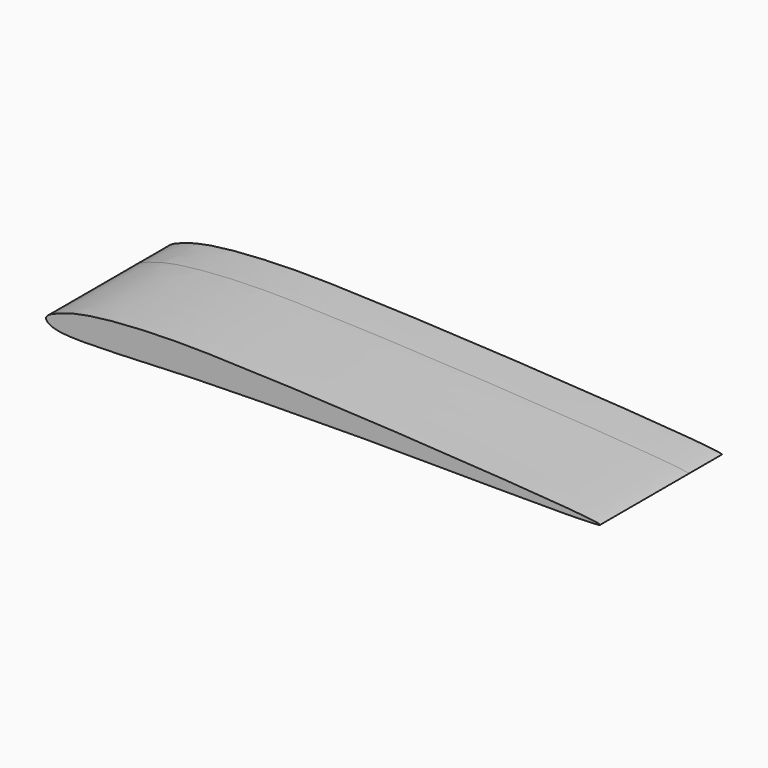
from build123d import *

# Parameters (mm, degrees)
F1_DEPTH = 20
F2_DEPTH = 7.5


with BuildPart() as f1:
    # F0 (on Front) → F1 (new body)
    with BuildSketch(Plane.XZ):
        with BuildLine():
            add(Edge.make_bspline(
                [(50.3091172778, -1.1656129636), (50.1718635236, -0.614292774), (8.6569150114, 1.9894121194), (-12.2185501878, 2.7626849393), (-26.6473375965, 3.249698923), (-38.2423795462, 2.6501887814), (-44.081300152, 1.7253239287), (-46.8139447574, 0.9123113702), (-50.2879633949, -0.4217517299), (-48.9166705509, -2.2301634685), (-42.4139489162, -2.6824339621), (-26.2734896509, -1.7533079921), (-8.3579730739, -1.4752937858), (13.4265681416, -1.2175639379), (50.4368833694, -1.6788231581), (50.3091172778, -1.1656129636)],
                knots=[0, 0, 0, 0, 0.1314800478, 0.240613753, 0.3188996978, 0.391566052, 0.4420501443, 0.4794543548, 0.5162860539, 0.5395368811, 0.5914550557, 0.6780096197, 0.7666368772, 0.8776085074, 1, 1, 1, 1], degree=3))
        make_face()
    extrude(amount=F1_DEPTH)

    # F0 (on Front) → F2 (join)
    with BuildSketch(Plane.XZ):
        with BuildLine():
            add(Edge.make_bspline(
                [(50.3091172778, -1.1656129636), (50.1718635236, -0.614292774), (8.6569150114, 1.9894121194), (-12.2185501878, 2.7626849393), (-26.6473375965, 3.249698923), (-38.2423795462, 2.6501887814), (-44.081300152, 1.7253239287), (-46.8139447574, 0.9123113702), (-50.2879633949, -0.4217517299), (-48.9166705509, -2.2301634685), (-42.4139489162, -2.6824339621), (-26.2734896509, -1.7533079921), (-8.3579730739, -1.4752937858), (13.4265681416, -1.2175639379), (50.4368833694, -1.6788231581), (50.3091172778, -1.1656129636)],
                knots=[0, 0, 0, 0, 0.1314800478, 0.240613753, 0.3188996978, 0.391566052, 0.4420501443, 0.4794543548, 0.5162860539, 0.5395368811, 0.5914550557, 0.6780096197, 0.7666368772, 0.8776085074, 1, 1, 1, 1], degree=3))
        make_face()
    extrude(amount=-F2_DEPTH)


solid = f1.part
